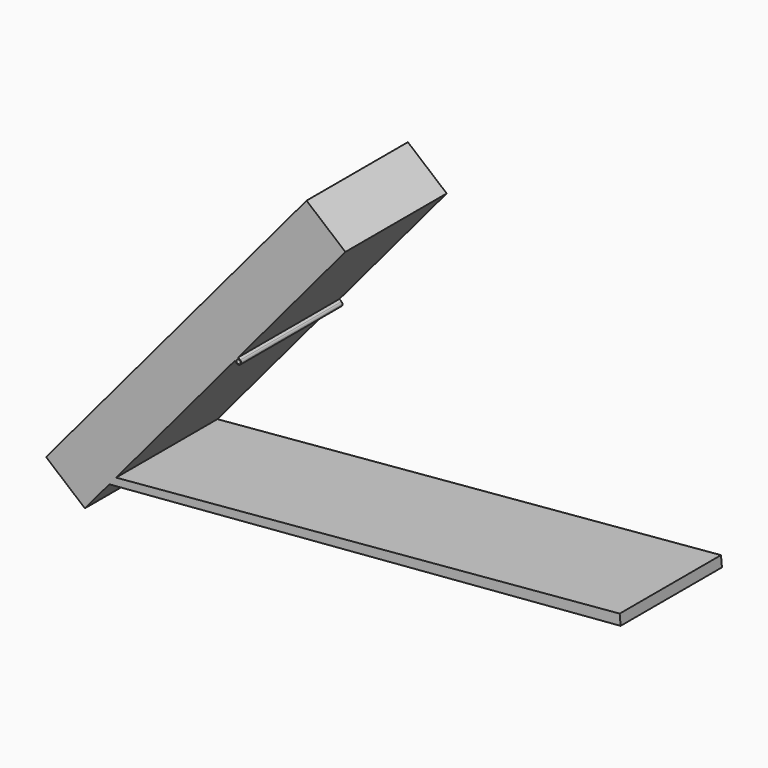
from build123d import *

# Parameters (mm, degrees)
F0_R     = 25.4
F1_DEPTH = 1524


# Not quite as in the source:
# - a feature names something its author has since deleted; it is built from what else it names


with BuildPart() as f1:
    # F0 (on Front) → F1 (new body)
    with BuildSketch(Plane.XZ):
        with BuildLine():
            Line((-2128.2773420369, 44.7304176766), (-838.4597244399, 1581.8751972391))
            Line((-838.4597244399, 1581.8751972391), (-1305.4404169652, 1973.718524104))
            Line((-1305.4404169652, 1973.718524104), (-4440.1870318845, -1762.1270160986))
            Line((-4440.1870318845, -1762.1270160986), (-3973.2063393592, -2153.9703429635))
            Line((-3973.2063393592, -2153.9703429635), (-3679.3238442105, -1803.7348235695))
            Line((-3679.3238442105, -1803.7348235695), (2473.8534732187, -1302.7410905921))
            Line((2473.8534732187, -1302.7410905921), (2462.7846938898, -1176.2243639345))
            Line((2462.7846938898, -1176.2243639345), (-3597.6898177803, -1706.4471792934))
            Line((-3597.6898177803, -1706.4471792934), (-2169.094355252, -3.9134044615))
            Line((-2169.094355252, -3.9134044615), (-2144.772444183, -24.321911069))
            ThreePointArc((-2144.772444183, -24.321911069), (-2100.0420265064, -20.4085066075), (-2103.9554309679, 24.321911069))
            Line((-2103.9554309679, 24.321911069), (-2128.2773420369, 44.7304176766))
        make_face()
        with Locations((-2124.3639375754, 0)):
            Circle(F0_R, mode=Mode.SUBTRACT)
    extrude(amount=F1_DEPTH)


solid = f1.part
